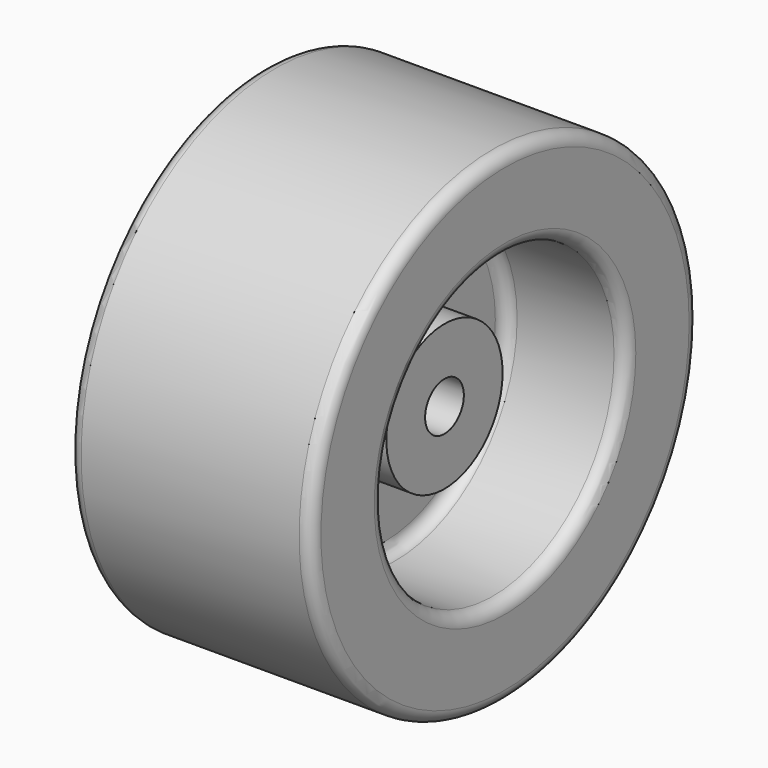
from build123d import *

# Parameters (mm, degrees)
F0_R     = 100
F1_DEPTH = 100
F2_R     = 5
F3_R     = 62.5
F4_DEPTH = 50
F5_R     = 30
F5_R_2   = 10
F6_DEPTH = 25
F7_R     = 5
F8_R     = 62.5
F9_DEPTH = 5
F10_R    = 2.49999


# Not quite as in the source:
# - a fillet or chamfer is up to 0.001 mm smaller than in the source, because OpenCascade refuses the exact size


with BuildPart() as f1:
    # F0 (on Right) → F1 (new body)
    with BuildSketch(Plane.YZ):
        Circle(F0_R)
    extrude(amount=F1_DEPTH)

    # F2
    f2_edges = [f1.edges().sort_by_distance(p)[0] for p in [
        (100, -100, 0),
        (0, -100, 0),
    ]]
    fillet(f2_edges, radius=F2_R)

    # F3 (on face) → F4 (cut)
    with BuildSketch(Plane.YZ.offset(100)):
        Circle(F3_R)
    extrude(amount=-F4_DEPTH, mode=Mode.SUBTRACT)

    # F5 (on face) → F6 (join)
    with BuildSketch(Plane.YZ.offset(50)):
        Circle(F5_R)
        Circle(F5_R_2, mode=Mode.SUBTRACT)
    extrude(amount=F6_DEPTH)

    # F7
    f7_edges = [f1.edges().sort_by_distance(p)[0] for p in [
        (50, -62.5, 0),
        (100, -62.5, 0),
        (50, -30, 0),
    ]]
    fillet(f7_edges, radius=F7_R)

    # F8 (on face) → F9 (cut)
    with BuildSketch(Plane(origin=(0, 0, 0), x_dir=(0, -1, 0), z_dir=(-1, 0, 0))):
        Circle(F8_R)
    extrude(amount=-F9_DEPTH, mode=Mode.SUBTRACT)

    # F10 (radius 2.5 in the source; OpenCascade refuses exactly that, so slightly less here)
    f10_edges = [f1.edges().sort_by_distance(p)[0] for p in [
        (0, 62.5, 0),
        (5, 62.5, 0),
    ]]
    fillet(f10_edges, radius=F10_R)


solid = f1.part
